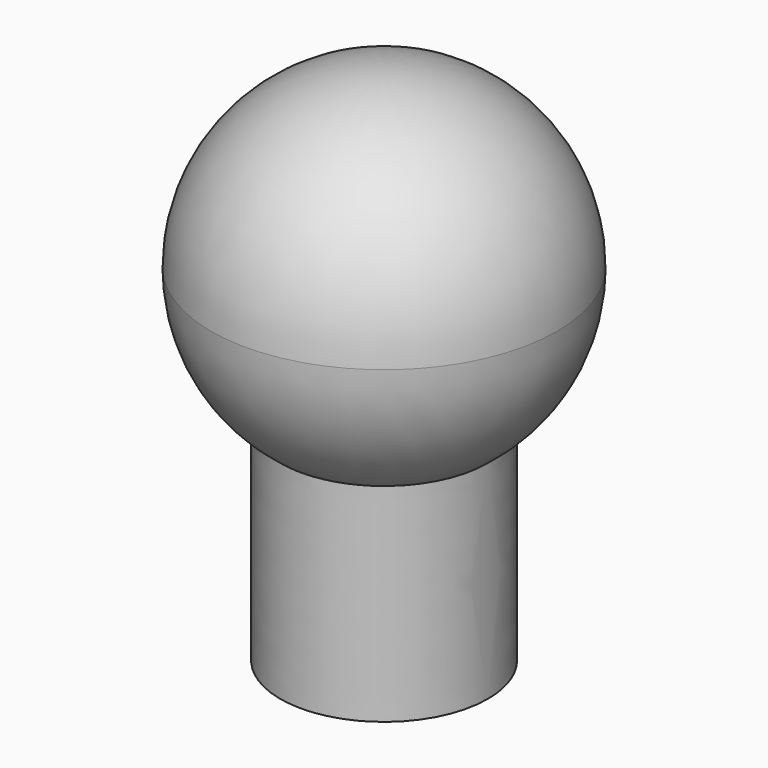
from build123d import *

# Parameters (mm, degrees)
F0_R     = 63.5
F1_DEPTH = 127
F2_R     = 63.49999
F3_DEPTH = 12.7
F4_DEPTH = 76.2
F5_T     = -2.54


# Not quite as in the source:
# - a fillet or chamfer is up to 0.001 mm smaller than in the source, because OpenCascade refuses the exact size


with BuildPart() as f1:
    # F0 (on Top) → F1 (new body)
    with BuildSketch(Plane.XY):
        Circle(F0_R)
    extrude(amount=F1_DEPTH)

    # F2 (radius 63.5 in the source; OpenCascade refuses exactly that, so slightly less here)
    f2_edges = [f1.edges().sort_by_distance(p)[0] for p in [
        (-63.5, 0, 127),
        (-63.5, 0, 0),
    ]]
    fillet(f2_edges, radius=F2_R)

    # F0 (on Top) → F3 (cut)
    with BuildSketch(Plane.XY):
        Circle(F0_R)
    extrude(amount=F3_DEPTH, mode=Mode.SUBTRACT)

    # F4 (add): a face of the model
    f4_faces = [f1.faces().sort_by_distance(p)[0] for p in [
        (-5.6883e-06, -3.51891e-05, 12.7),
    ]]
    extrude(f4_faces, amount=F4_DEPTH)

    # F5
    f5_openings = [f1.faces().sort_by_distance(p)[0] for p in [
        (-6e-06, -3.5e-05, -63.5),
    ]]
    offset(amount=F5_T, openings=f5_openings, kind=Kind.INTERSECTION)


solid = f1.part
